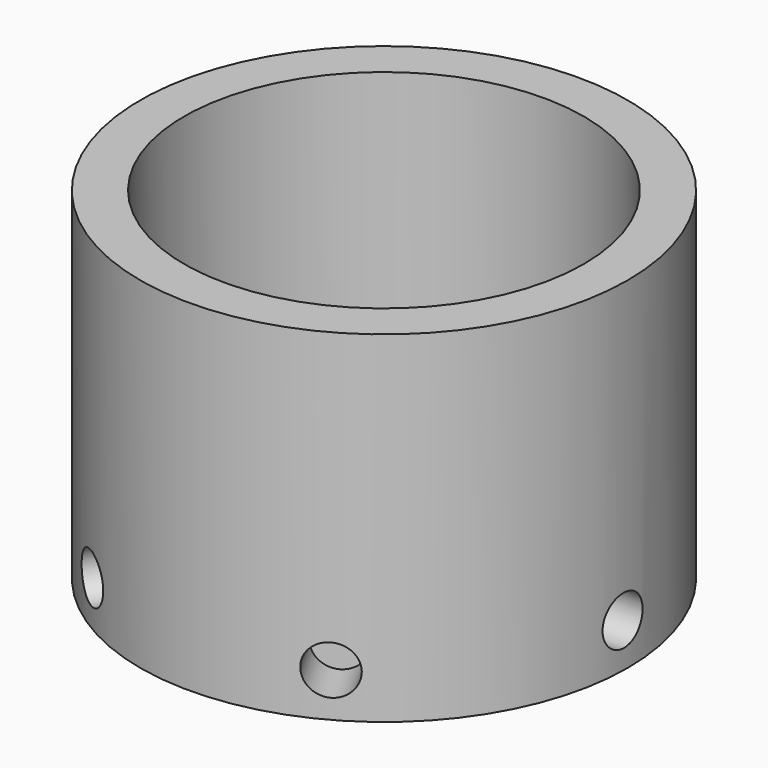
from build123d import *

# Parameters (mm, degrees)
F0_R             = 25
F1_DEPTH         = 35
F2_R             = 20.5
F3_DEPTH         = 27
F4_R             = 7.5
F5_DEPTH         = 8.001
F6_R             = 13.5
F7_DEPTH         = 2
F10_R            = 2.5
F11_DEPTH        = 5
F11_COPIES_COUNT = 6


# Not quite as in the source:
# - a pattern or mirror of a feature is missing from the dataset's text; its kind, count and spacing are read off the source's solid


with BuildPart() as f1:
    # F0 (on Top) → F1 (new body)
    with BuildSketch(Plane.XY):
        with Locations((0, 6.5720938146)):
            Circle(F0_R)
    extrude(amount=F1_DEPTH)

    # F2 (on face) → F3 (cut)
    with BuildSketch(Plane.XY.offset(35)):
        with Locations((0, 6.5720938146)):
            Circle(F2_R)
    extrude(amount=-F3_DEPTH, mode=Mode.SUBTRACT)

    # F4 (on face) → F5 (cut, through all)
    with BuildSketch(Plane.XY.offset(8)):
        with Locations((0, 6.5720938146)):
            Circle(F4_R)
    extrude(amount=-F5_DEPTH, mode=Mode.SUBTRACT)

    # F6 (on face) → F7 (cut)
    with BuildSketch(Plane.XY.offset(8)):
        with Locations((0, 6.5720938146)):
            Circle(F6_R)
    extrude(amount=-F7_DEPTH, mode=Mode.SUBTRACT)

    # F10 (on offset) → F11 (cut)
    with BuildSketch(Plane.YZ.offset(25)):
        with Locations((6.071, 4.5)):
            Circle(F10_R)
    f11 = extrude(amount=-F11_DEPTH, mode=Mode.SUBTRACT)

    # F11_copies: F11 ×6 about axis
    f11_copies_axis = Axis((0, 6.572094, 0), (0, 0, 1))
    for i in range(1, F11_COPIES_COUNT):
        add(f11.rotate(f11_copies_axis, i * 360 / F11_COPIES_COUNT), mode=Mode.SUBTRACT)


solid = f1.part
